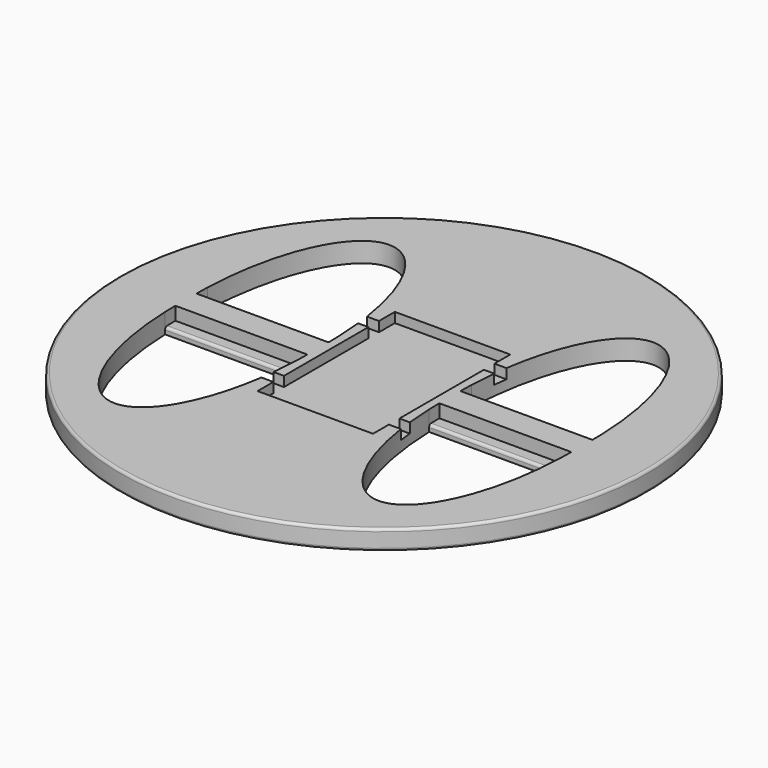
from build123d import *

# Parameters (mm, degrees)
F1_DEPTH = 19.05
F2_DEPTH = 6.35
F4_R     = 2.54
F5_START = 9.525
F3_W     = 111.125
F3_H     = 19.05
F3_H_2   = 12.7
F3_W_2   = 46.0375
F5_DEPTH = 9.525


# Not quite as in the source:
# - two fillets or chamfers of one size are made in one step


with BuildPart() as f1:
    # F0 (on Top) → F1 (new body)
    with BuildSketch(Plane.XY):
        with BuildLine():
            Line((0, 0), (254, 0))
            ThreePointArc((254, 0), (179.6051224214, 179.6051224214), (0, 254))
            Line((0, 254), (0, 0))
        make_face()
        with BuildLine():
            add(Edge.make_bspline(
                [(190.5, 12.7), (190.5, 19.0610627513), (190.2791297656, 25.4)],
                knots=[1.5707963268, 1.5707963268, 1.5707963268, 1.6542264134, 1.6542264134, 1.6542264134], degree=2, weights=[1, 0.9991300537, 1]))
            Line((190.5, 12.7), (63.5, 12.7))
            add(Edge.make_bspline(
                [(63.7208702344, 25.4), (63.5, 19.0610627513), (63.5, 12.7)],
                knots=[4.6289588938, 4.6289588938, 4.6289588938, 4.7123889804, 4.7123889804, 4.7123889804], degree=2, weights=[1, 0.9991300537, 1]))
            add(Edge.make_bspline(
                [(190.2791297656, 25.4), (185.411504399, 165.1), (127, 165.1), (68.588495601, 165.1), (63.7208702344, 25.4)],
                knots=[1.6542264134, 1.6542264134, 1.6542264134, 3.1415926536, 3.1415926536, 4.6289588938, 4.6289588938, 4.6289588938], degree=2, weights=[1, 0.7359800722, 1, 0.7359800722, 1]))
        make_face(mode=Mode.SUBTRACT)
        with BuildLine():
            ThreePointArc((0, -254), (179.6051224214, -179.6051224214), (254, 0))
            Line((254, 0), (0, 0))
            Line((0, 0), (0, -254))
        make_face()
        with BuildLine():
            add(Edge.make_bspline(
                [(63.5, -12.7), (63.5, -19.0610627513), (63.7208702344, -25.4)],
                knots=[1.5707963268, 1.5707963268, 1.5707963268, 1.6542264134, 1.6542264134, 1.6542264134], degree=2, weights=[1, 0.9991300537, 1]))
            Line((63.5, -12.7), (190.5, -12.7))
            add(Edge.make_bspline(
                [(190.2791297656, -25.4), (190.5, -19.0610627513), (190.5, -12.7)],
                knots=[4.6289588938, 4.6289588938, 4.6289588938, 4.7123889804, 4.7123889804, 4.7123889804], degree=2, weights=[1, 0.9991300537, 1]))
            add(Edge.make_bspline(
                [(63.7208702344, -25.4), (68.588495601, -165.1), (127, -165.1), (185.411504399, -165.1), (190.2791297656, -25.4)],
                knots=[1.6542264134, 1.6542264134, 1.6542264134, 3.1415926536, 3.1415926536, 4.6289588938, 4.6289588938, 4.6289588938], degree=2, weights=[1, 0.7359800722, 1, 0.7359800722, 1]))
        make_face(mode=Mode.SUBTRACT)
        with BuildLine():
            Line((0, 0), (0, 254))
            ThreePointArc((0, 254), (-179.6051224214, 179.6051224214), (-254, 0))
            Line((-254, 0), (0, 0))
        make_face()
        with BuildLine():
            add(Edge.make_bspline(
                [(-63.5, 12.7), (-63.5, 19.0610627513), (-63.7208702344, 25.4)],
                knots=[1.5707963268, 1.5707963268, 1.5707963268, 1.6542264134, 1.6542264134, 1.6542264134], degree=2, weights=[1, 0.9991300537, 1]))
            Line((-63.5, 12.7), (-190.5, 12.7))
            add(Edge.make_bspline(
                [(-190.2791297656, 25.4), (-190.5, 19.0610627513), (-190.5, 12.7)],
                knots=[4.6289588938, 4.6289588938, 4.6289588938, 4.7123889804, 4.7123889804, 4.7123889804], degree=2, weights=[1, 0.9991300537, 1]))
            add(Edge.make_bspline(
                [(-63.7208702344, 25.4), (-68.588495601, 165.1), (-127, 165.1), (-185.411504399, 165.1), (-190.2791297656, 25.4)],
                knots=[1.6542264134, 1.6542264134, 1.6542264134, 3.1415926536, 3.1415926536, 4.6289588938, 4.6289588938, 4.6289588938], degree=2, weights=[1, 0.7359800722, 1, 0.7359800722, 1]))
        make_face(mode=Mode.SUBTRACT)
        with BuildLine():
            ThreePointArc((-254, 0), (-179.6051224214, -179.6051224214), (0, -254))
            Line((0, -254), (0, 0))
            Line((0, 0), (-254, 0))
        make_face()
        with BuildLine():
            add(Edge.make_bspline(
                [(-190.5, -12.7), (-190.5, -19.0610627513), (-190.2791297656, -25.4)],
                knots=[1.5707963268, 1.5707963268, 1.5707963268, 1.6542264134, 1.6542264134, 1.6542264134], degree=2, weights=[1, 0.9991300537, 1]))
            Line((-190.5, -12.7), (-63.5, -12.7))
            add(Edge.make_bspline(
                [(-63.7208702344, -25.4), (-63.5, -19.0610627513), (-63.5, -12.7)],
                knots=[4.6289588938, 4.6289588938, 4.6289588938, 4.7123889804, 4.7123889804, 4.7123889804], degree=2, weights=[1, 0.9991300537, 1]))
            add(Edge.make_bspline(
                [(-190.2791297656, -25.4), (-185.411504399, -165.1), (-127, -165.1), (-68.588495601, -165.1), (-63.7208702344, -25.4)],
                knots=[1.6542264134, 1.6542264134, 1.6542264134, 3.1415926536, 3.1415926536, 4.6289588938, 4.6289588938, 4.6289588938], degree=2, weights=[1, 0.7359800722, 1, 0.7359800722, 1]))
        make_face(mode=Mode.SUBTRACT)
    extrude(amount=F1_DEPTH)

    # F0 (on Top) → F2 (join)
    with BuildSketch(Plane.XY):
        with BuildLine():
            Line((63.5, 12.7), (190.5, 12.7))
            add(Edge.make_bspline(
                [(190.5, 12.7), (190.5, 19.0610627513), (190.2791297656, 25.4)],
                knots=[1.5707963268, 1.5707963268, 1.5707963268, 1.6542264134, 1.6542264134, 1.6542264134], degree=2, weights=[1, 0.9991300537, 1]))
            Line((190.2791297656, 25.4), (63.7208702344, 25.4))
            add(Edge.make_bspline(
                [(63.7208702344, 25.4), (63.5, 19.0610627513), (63.5, 12.7)],
                knots=[4.6289588938, 4.6289588938, 4.6289588938, 4.7123889804, 4.7123889804, 4.7123889804], degree=2, weights=[1, 0.9991300537, 1]))
        make_face()
        with BuildLine():
            Line((190.5, -12.7), (63.5, -12.7))
            add(Edge.make_bspline(
                [(63.5, -12.7), (63.5, -19.0610627513), (63.7208702344, -25.4)],
                knots=[1.5707963268, 1.5707963268, 1.5707963268, 1.6542264134, 1.6542264134, 1.6542264134], degree=2, weights=[1, 0.9991300537, 1]))
            Line((63.7208702344, -25.4), (190.2791297656, -25.4))
            add(Edge.make_bspline(
                [(190.2791297656, -25.4), (190.5, -19.0610627513), (190.5, -12.7)],
                knots=[4.6289588938, 4.6289588938, 4.6289588938, 4.7123889804, 4.7123889804, 4.7123889804], degree=2, weights=[1, 0.9991300537, 1]))
        make_face()
        with BuildLine():
            Line((-63.5, -12.7), (-190.5, -12.7))
            add(Edge.make_bspline(
                [(-190.5, -12.7), (-190.5, -19.0610627513), (-190.2791297656, -25.4)],
                knots=[1.5707963268, 1.5707963268, 1.5707963268, 1.6542264134, 1.6542264134, 1.6542264134], degree=2, weights=[1, 0.9991300537, 1]))
            Line((-190.2791297656, -25.4), (-63.7208702344, -25.4))
            add(Edge.make_bspline(
                [(-63.7208702344, -25.4), (-63.5, -19.0610627513), (-63.5, -12.7)],
                knots=[4.6289588938, 4.6289588938, 4.6289588938, 4.7123889804, 4.7123889804, 4.7123889804], degree=2, weights=[1, 0.9991300537, 1]))
        make_face()
        with BuildLine():
            Line((-190.5, 12.7), (-63.5, 12.7))
            add(Edge.make_bspline(
                [(-63.5, 12.7), (-63.5, 19.0610627513), (-63.7208702344, 25.4)],
                knots=[1.5707963268, 1.5707963268, 1.5707963268, 1.6542264134, 1.6542264134, 1.6542264134], degree=2, weights=[1, 0.9991300537, 1]))
            Line((-63.7208702344, 25.4), (-190.2791297656, 25.4))
            add(Edge.make_bspline(
                [(-190.2791297656, 25.4), (-190.5, 19.0610627513), (-190.5, 12.7)],
                knots=[4.6289588938, 4.6289588938, 4.6289588938, 4.7123889804, 4.7123889804, 4.7123889804], degree=2, weights=[1, 0.9991300537, 1]))
        make_face()
    extrude(amount=F2_DEPTH)

    # F4
    f4_edges = [f1.edges().sort_by_distance(p)[0] for p in [
        (254, 0, 19.05),
        (-127, -25.4, 6.35),
        (127, -25.4, 6.35),
        (127, 25.4, 6.35),
        (-127, 25.4, 6.35),
        (254, 0, 0),
    ]]
    fillet(f4_edges, radius=F4_R)

    # F3 (on Top) → F5 (cut)
    with BuildSketch(Plane.XY.offset(F5_START)):
        with Locations((0, 73.025)):
            Rectangle(F3_W, F3_H)
        with Locations((0, 57.15)):
            Rectangle(F3_W, F3_H_2)
        with Locations((-78.58125, 57.15)):
            Rectangle(F3_W_2, F3_H_2)
        with Locations((78.58125, 57.15)):
            Rectangle(F3_W_2, F3_H_2)
        Polygon((55.5625, 50.8), (-55.5625, 50.8), (-55.5625, -50.8), (55.5625, -50.8), (55.5625, 0), align=None)
        with Locations((0, -57.15)):
            Rectangle(F3_W, F3_H_2)
        with Locations((-78.58125, -57.15)):
            Rectangle(F3_W_2, F3_H_2)
        with Locations((0, -73.025)):
            Rectangle(F3_W, F3_H)
        with Locations((78.58125, -57.15)):
            Rectangle(F3_W_2, F3_H_2)
    extrude(amount=F5_DEPTH, mode=Mode.SUBTRACT)


solid = f1.part
